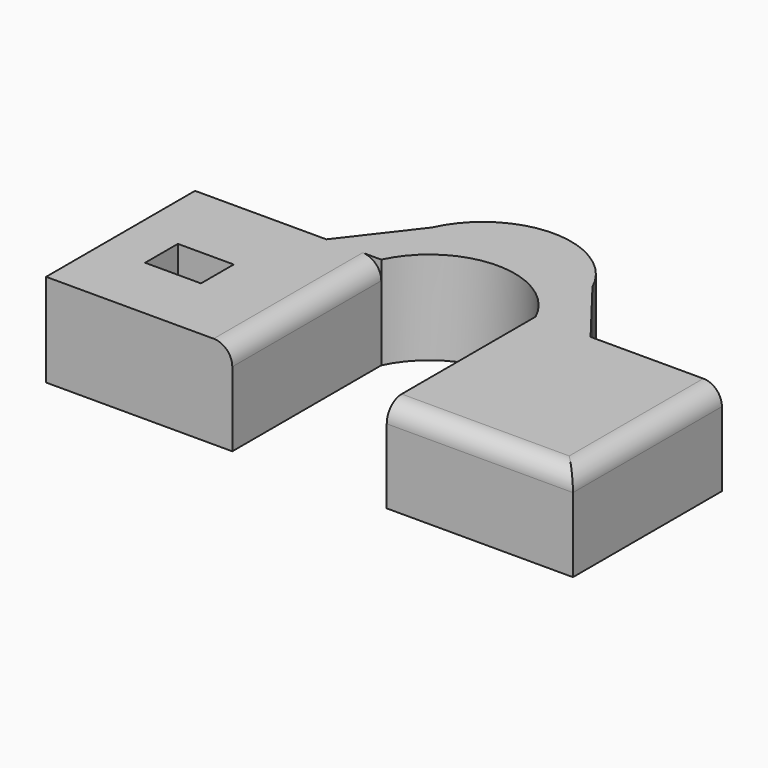
from build123d import *

# Parameters (mm, degrees)
F0_W     = 50
F0_H     = 25
F1_DEPTH = 50
F2_R     = 5
F2_2_R   = 5
F3_W     = 15
F3_H     = 11
F3_R     = 5
F4_DEPTH = 8
F7_DEPTH = 25


with BuildPart() as f1:
    # F0 (on Front) → F1 (new body)
    with BuildSketch(Plane.XZ):
        with Locations((51.8986206502, 45.4651199281)):
            Rectangle(F0_W, F0_H)
    extrude(amount=F1_DEPTH)

    # F2
    f2_edges = [f1.edges().sort_by_distance(p)[0] for p in [
        (76.898621, -25, 57.96512),
    ]]
    fillet(f2_edges, radius=F2_R)

    # F3 (on face) → F4 (cut)
    with BuildSketch(Plane.XY.offset(57.9651199281)):
        with Locations((46.6270151734, -26.549421221)):
            Rectangle(F3_W, F3_H)
        with Locations((140.8739293367, -25.6193820387)):
            Circle(F3_R)
    extrude(amount=-F4_DEPTH, mode=Mode.SUBTRACT)



with BuildPart() as f1b:
    # F0 (on Front) → F1, piece 2 (new body)
    with BuildSketch(Plane.XZ):
        with Locations((143.3739293367, 45.4651199281)):
            Rectangle(F0_W, F0_H)
    extrude(amount=F1_DEPTH)

    # F2#2
    f2_2_edges = [f1b.edges().sort_by_distance(p)[0] for p in [
        (168.373929, -25, 57.96512),
        (143.373929, -50, 57.96512),
    ]]
    fillet(f2_2_edges, radius=F2_2_R)


with BuildPart() as f1_1:
    add(f1.part)

    add(f1b.part)  # F7 merges F1b
    # F6 (on offset) → F7 (join)
    with BuildSketch(Plane(origin=(0, 0, 32.9651199281), x_dir=(1, 0, 0), z_dir=(0, 0, -1))):
        with BuildLine():
            ThreePointArc((118.3739293367, 0), (97.6362749934, -13.1297755552), (76.8986206502, 0))
            Line((76.8986206502, 0), (62.1641688049, 0))
            Line((62.1641688049, 0), (76.054610312, -17.9887413979))
            ThreePointArc((76.054610312, -17.9887413979), (97.6362749934, -31.8841869417), (119.2179396749, -17.9887413979))
            Line((119.2179396749, -17.9887413979), (133.108381182, 0))
            Line((133.108381182, 0), (118.3739293367, 0))
        make_face()
    extrude(amount=-F7_DEPTH)


solid = f1_1.part
